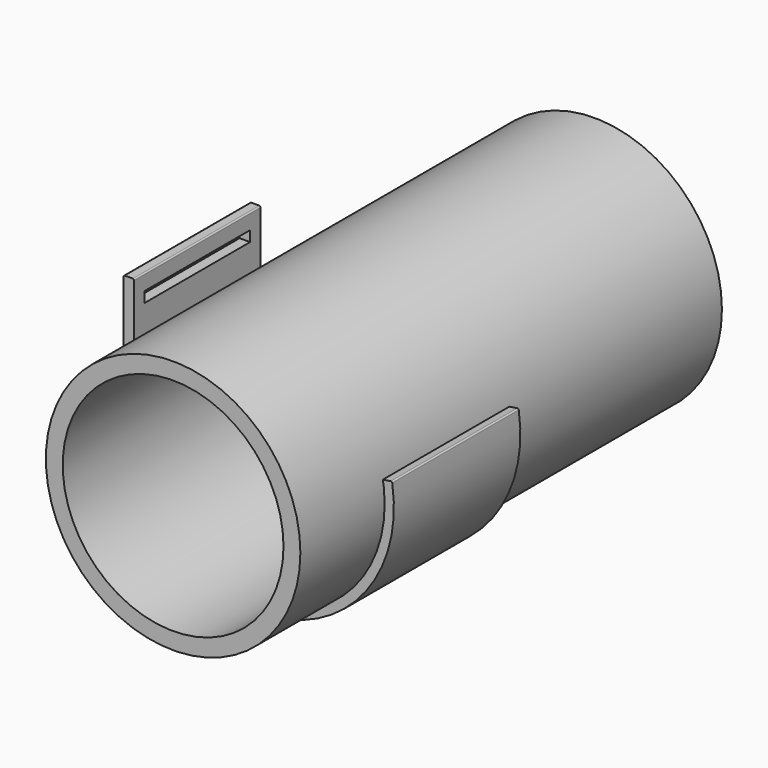
from build123d import *

# Parameters (mm, degrees)
F0_R     = 24.15
F0_R_2   = 20.95
F1_DEPTH = 50
F3_DEPTH = 30
F5_W     = 25
F5_H     = 2
F6_DEPTH = 51.2881315685


# Not quite as in the source:
# - a feature of the source that left no trace in its solid (it failed there, or was rolled back) is left out


with BuildPart() as f1:
    # F0 (on Front) → F1 (new body, symmetric)
    with BuildSketch(Plane.XZ):
        Circle(F0_R)
        Circle(F0_R_2, mode=Mode.SUBTRACT)
    extrude(amount=F1_DEPTH, both=True)


with BuildPart() as f3:
    # F2 (on Front) → F3 (new body)
    with BuildSketch(Plane.XZ):
        with BuildLine():
            Line((-25.3868595608, 21.8855109754), (-25.3868595608, 6.0457583589))
            ThreePointArc((-25.3868595608, 6.0457583589), (-25.4275675824, 5.1443687165), (-25.5493602183, 4.250317832))
            ThreePointArc((-25.5493602183, 4.250317832), (-0.1257323753, -25.8986821176), (25.5894092407, 4.0020627281))
            ThreePointArc((25.5894092407, 4.0020627281), (25.4891661105, 4.1658377534), (25.3023462898, 4.2102145337))
            Line((25.3023462898, 4.2102145337), (23.8321379738, 3.9715227194))
            ThreePointArc((23.8321379738, 3.9715227194), (23.6698358356, 3.8715466122), (23.6251881424, 3.6862258374))
            ThreePointArc((23.6251881424, 3.6862258374), (-0.1242226088, -23.9092333702), (-23.5856250226, 3.9315007559))
            ThreePointArc((-23.5856250226, 3.9315007559), (-23.4366750052, 4.9184773412), (-23.3868595608, 5.9153862181))
            Line((-23.3868595608, 5.9153862181), (-23.3868595608, 21.8855109754))
            ThreePointArc((-23.3868595608, 21.8855109754), (-23.4600828655, 22.0622876707), (-23.6368595608, 22.1355109754))
            Line((-23.6368595608, 22.1355109754), (-25.1368595608, 22.1355109754))
            ThreePointArc((-25.1368595608, 22.1355109754), (-25.3136362561, 22.0622876707), (-25.3868595608, 21.8855109754))
        make_face()
    extrude(amount=F3_DEPTH)

    # F5 (on face) → F6 (cut, through all)
    with BuildSketch(Plane(origin=(-25.3868595608, 0, 0), x_dir=(0, -1, 0), z_dir=(-1, 0, 0))):
        with Locations((15, 18.1355109754)):
            Rectangle(F5_W, F5_H)
    extrude(amount=-F6_DEPTH, mode=Mode.SUBTRACT)


solid = Compound([f1.part, f3.part])
